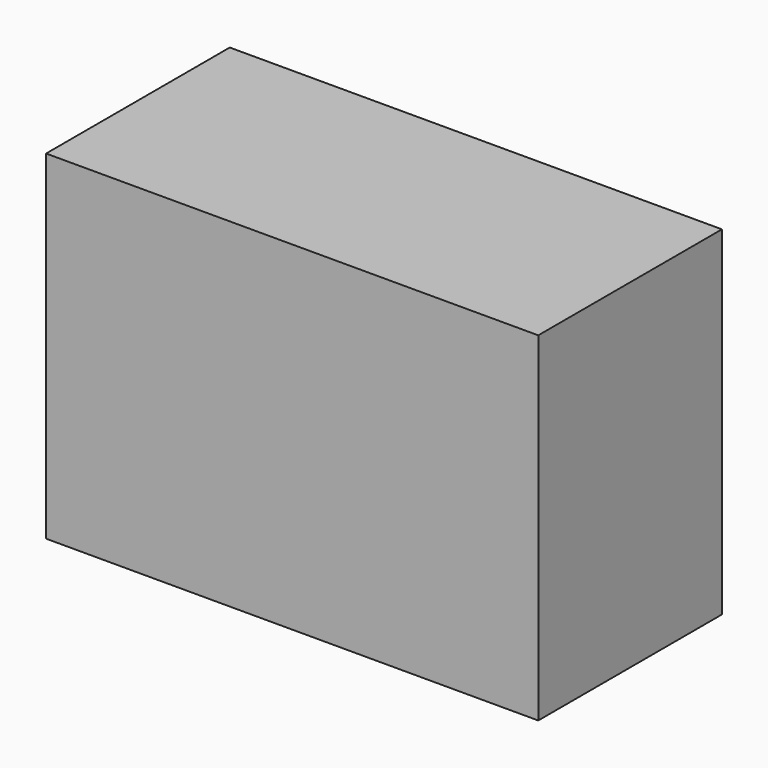
from build123d import *

# Parameters (mm, degrees)
F0_W     = 53.5966232419
F0_H     = 36.9254415855
F1_DEPTH = 25


# Not quite as in the source:
# - the program builds the solid bodies; features that only make, move or delete a surface that nothing else refers to are left out


with BuildPart() as f1:
    # F0 (on Front) → F1 (new body)
    with BuildSketch(Plane.XZ):
        with Locations((-53.0379377306, 9.0313074179)):
            Rectangle(F0_W, F0_H)
    extrude(amount=F1_DEPTH)


solid = f1.part
